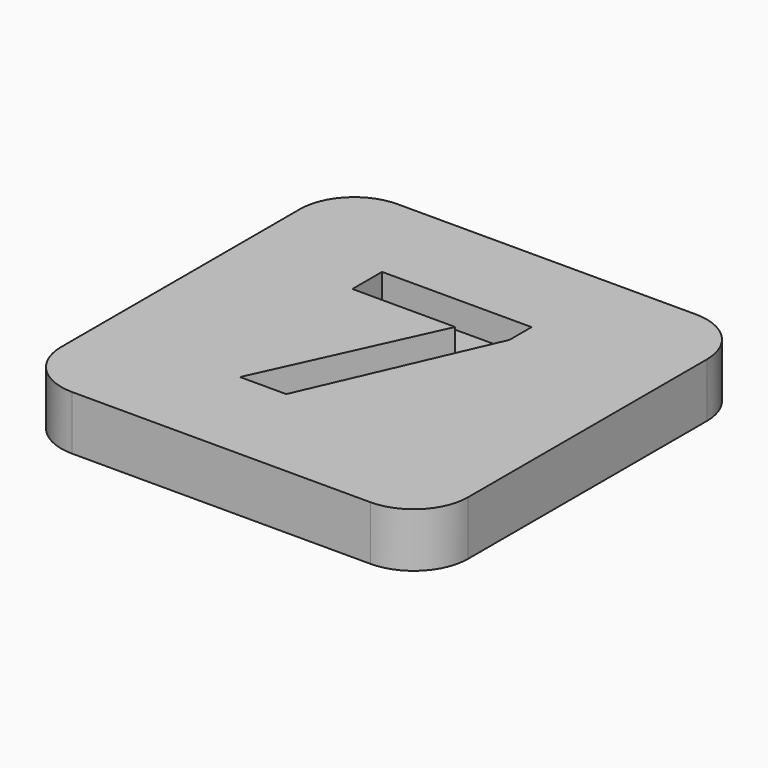
from build123d import *

# Parameters (mm, degrees)
F0_W         = 38.1
F0_H         = 38.1
F1_DEPTH     = 5.08
F2_TEXT_SIZE = 27.3386804657
F3_DEPTH     = 2.54
F4_R         = 5.08


# Not quite as in the source:
# - Text() gives the source's letters only with a copy of the font that has no kerning and outlines rounded to 1/6400 em; it was checked with that copy


with BuildPart() as f1:
    # F0 (on Top) → F1 (new body)
    with BuildSketch(Plane.XY):
        Rectangle(F0_W, F0_H)
    extrude(amount=F1_DEPTH)

    # F2 (on face) → F3 (cut)
    with BuildSketch(Plane.XY.offset(5.08)):
        with Locations((-8.89, -9.525)):
            Text('7', F2_TEXT_SIZE, font='Open Sans', font_style=FontStyle.BOLD, text_align=(TextAlign.LEFT, TextAlign.BOTTOM))
    extrude(amount=-F3_DEPTH, mode=Mode.SUBTRACT)

    # F4
    f4_edges = [f1.edges().sort_by_distance(p)[0] for p in [
        (-19.05, -19.05, 2.54),
        (19.05, -19.05, 2.54),
        (19.05, 19.05, 2.54),
        (-19.05, 19.05, 2.54),
    ]]
    fillet(f4_edges, radius=F4_R)


solid = f1.part
